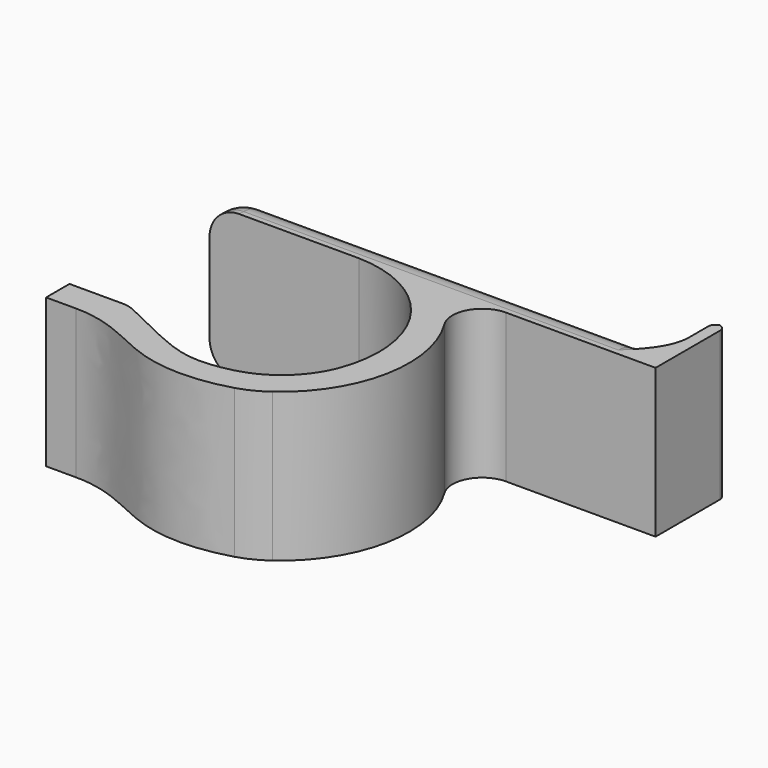
from build123d import *

# Parameters (mm, degrees)
F1_DEPTH     = 25.4
F2_R         = 5.08
F3_T1_DEPTH  = 15.24
F3_T6_ANGLE  = 233.2969892374
F3_T12_ANGLE = 233.2969892374
F4_T1_DEPTH  = 31.75
F5_R         = 15.24
F6_R         = 5.08
F7_R         = 5.08
F8_R         = 5.08


# Not quite as in the source:
# - a fillet or chamfer that OpenCascade refuses, or shapes differently, is made with other operations: its cross-section is extruded or revolved along the edge and cut away or added


with BuildPart() as f1:
    # F0 (on Top) → F1 (new body)
    with BuildSketch(Plane.XY):
        Polygon((0, 6), (0, 0), (25.5269114748, 0), (38.1, 0), (76.2, 0), (76.2, 15), (74.2, 15), (74.2, 6), align=None)
        with BuildLine():
            Line((38.1, 0), (25.5269114748, 0))
            ThreePointArc((25.5269114748, 0), (43.3170296074, -12.6890998813), (38.1, -33.909))
            add(Edge.make_bspline(
                [(10.1822623983, -29.9098208), (13.5454405981, -31.48996992), (21.4109886211, -35.5910719416), (28.6130215973, -37.6913323998), (38.1, -33.909)],
                knots=[0, 0, 0, 0, 0.4439990675, 1, 1, 1, 1], degree=3))
            Line((10.1822623983, -29.9098208), (0, -29.9098208))
            Line((0, -29.9098208), (0, -34.9098208))
            Line((0, -34.9098208), (5.0913545239, -34.9098208))
            add(Edge.make_bspline(
                [(38.1, -38.909), (31.7124112149, -41.2898788749), (19.626955474, -41.5346198852), (11.6216761715, -34.9098208), (5.0913545239, -34.9098208)],
                knots=[0, 0, 0, 0, 0.512363552, 1, 1, 1, 1], degree=3))
            ThreePointArc((38.1, -38.909), (49.6761075901, -19.4545), (38.1, 0))
        make_face()
    extrude(amount=F1_DEPTH)

    # F2
    f2_edges = [f1.edges().sort_by_distance(p)[0] for p in [
        (37.1, 6, 25.4),
        (37.1, 6, 0),
    ]]
    fillet(f2_edges, radius=F2_R)

    # F3: fillet of radius 5.08 on 1 edges, made by hand

    # F3_s2 → F3_t1 (join)
    with BuildSketch(Plane.XY.offset(5.08)):
        with BuildLine():
            ThreePointArc((69.12, 6), (72.7121024484, 7.4878975516), (74.2, 11.08))
            Line((74.2, 11.08), (74.2, 6))
            Line((74.2, 6), (69.12, 6))
        make_face()
    extrude(amount=F3_T1_DEPTH)


with BuildPart() as f3_tool4:
    # F3_s5 → F3_t6 (revolve)
    with BuildSketch(Plane.XY.offset(5.08)):
        with BuildLine():
            ThreePointArc((69.12, 6), (72.7121024484, 7.4878975516), (74.2, 11.08))
            Line((74.2, 11.08), (74.2, 6))
            Line((74.2, 6), (69.12, 6))
        make_face()
    revolve(axis=Axis((74.2, 0.92, 5.08), (-1, 0, 0)), revolution_arc=F3_T6_ANGLE)

    split(bisect_by=Plane.XY, keep=Keep.TOP)

    split(bisect_by=Plane.XZ, keep=Keep.BOTTOM)


with BuildPart() as f1_1:
    add(f1.part)

    # F3_t3: union F3_tool4
    add(f3_tool4.part)


with BuildPart() as f3_tool10:
    # F3_s11 → F3_t12 (revolve)
    with BuildSketch(Plane.XY.offset(20.32)):
        with BuildLine():
            ThreePointArc((69.12, 6), (72.7121024484, 7.4878975516), (74.2, 11.08))
            Line((74.2, 11.08), (74.2, 6))
            Line((74.2, 6), (69.12, 6))
        make_face()
    revolve(axis=Axis((74.2, 0.92, 20.32), (1, 0, 0)), revolution_arc=F3_T12_ANGLE)

    split(bisect_by=Plane.XY.offset(25.4), keep=Keep.BOTTOM)

    split(bisect_by=Plane.XZ, keep=Keep.BOTTOM)


with BuildPart() as f1_2:
    add(f1_1.part)

    # F3_t9: union F3_tool10
    add(f3_tool10.part)

    # F4: fillet of radius 1.27 on 2 edges, made by hand

    # F4_s2 → F4_t1 (cut)
    with BuildSketch(Plane.XY.offset(-3.175)):
        with BuildLine():
            ThreePointArc((75.47, 15), (74.5719743879, 14.6280256121), (74.2, 13.73))
            Line((74.2, 13.73), (74.2, 15))
            Line((74.2, 15), (75.47, 15))
        make_face()
        with BuildLine():
            ThreePointArc((76.2, 13.73), (75.8280256121, 14.6280256121), (74.93, 15))
            Line((74.93, 15), (76.2, 15))
            Line((76.2, 15), (76.2, 13.73))
        make_face()
    extrude(amount=F4_T1_DEPTH, mode=Mode.SUBTRACT)

    # F5
    f5_edges = [f1_2.edges().sort_by_distance(p)[0] for p in [
        (38.1, -38.909, 12.7),
        (38.1, -33.909, 12.7),
    ]]
    fillet(f5_edges, radius=F5_R)

    # F6
    f6_edges = [f1_2.edges().sort_by_distance(p)[0] for p in [
        (38.1, 0, 12.7),
    ]]
    fillet(f6_edges, radius=F6_R)

    # F7
    f7_edges = [f1_2.edges().sort_by_distance(p)[0] for p in [
        (10.182262, -29.909821, 12.7),
    ]]
    fillet(f7_edges, radius=F7_R)

    # F8
    f8_edges = [f1_2.edges().sort_by_distance(p)[0] for p in [
        (0, 6, 12.7),
        (0, 0.46, 0),
        (0, 4.512102, 1.487898),
        (0, 4.512102, 23.912102),
        (0, 0.46, 25.4),
    ]]
    fillet(f8_edges, radius=F8_R)


solid = f1_2.part
